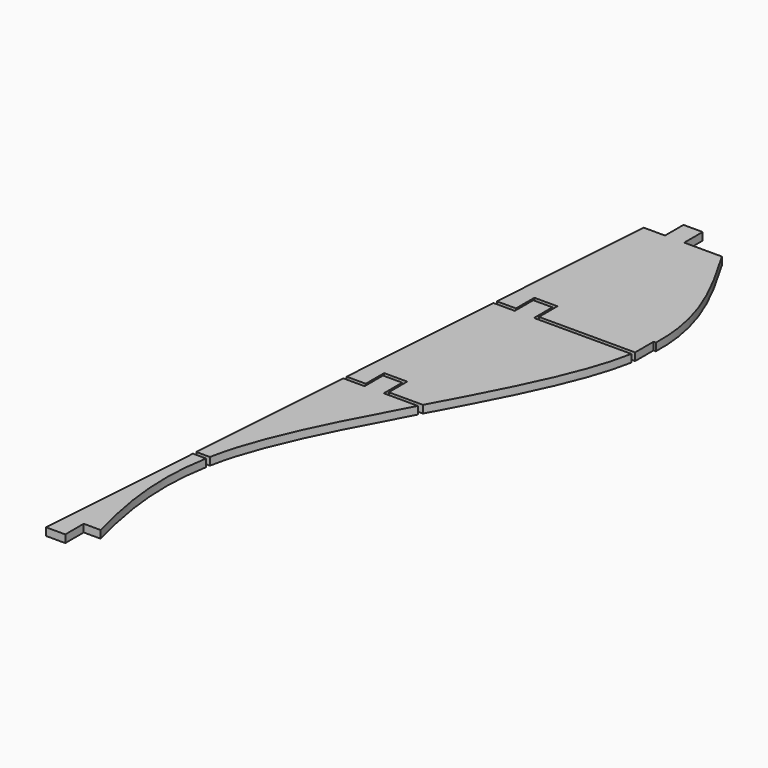
from build123d import *

# Parameters (mm, degrees)
F1_DEPTH = 2


with BuildPart() as f1:
    # F0 (on Top) → F1 (new body)
    with BuildSketch(Plane.XY):
        with BuildLine():
            Line((-20.4571957112, 87.1), (-23.5168766766, 43.1))
            Line((-23.5168766766, 43.1), (-18.5168766766, 43.1))
            Line((-18.5168766766, 43.1), (-18.5168766766, 49.1))
            Line((-18.5168766766, 49.1), (-12.5168766766, 49.1))
            Line((-12.5168766766, 49.1), (-12.5168766766, 43.1))
            Line((-12.5168766766, 43.1), (12.5168766766, 43.1))
            Line((12.5168766766, 43.1), (12.5168766766, 49.1))
            Line((12.5168766766, 49.1), (13.1200117893, 49.0999999996))
            add(Edge.make_bspline(
                [(-0.0691957112, 87.1), (6.7670600664, 75.385477326), (13.603315844, 63.6709546521), (13.1200117893, 49.0999999996)],
                knots=[0, 0, 0, 0, 0.2539558406, 0.2539558406, 0.2539558406, 0.2539558406], degree=3))
            Line((-0.0691957112, 87.1), (-9.8876575074, 87.1))
            Line((-9.8876575074, 87.1), (-9.8876575074, 93.1))
            Line((-9.8876575074, 93.1), (-14.8876575074, 93.1))
            Line((-14.8876575074, 93.1), (-14.8876575074, 87.1))
            Line((-14.8876575074, 87.1), (-20.4571957112, 87.1))
        make_face()
    extrude(amount=F1_DEPTH)


with BuildPart() as f1b:
    # F0 (on Top) → F1, piece 2 (new body)
    with BuildSketch(Plane.XY):
        with BuildLine():
            add(Edge.make_bspline(
                [(-26.4305470242, -47.9), (-28.9813165577, -61.9153804796), (-26.6038291609, -74.0441530198), (-23.513396984, -85.9)],
                knots=[0.7330193554, 0.7330193554, 0.7330193554, 0.7330193554, 0.9613773268, 0.9613773268, 0.9613773268, 0.9613773268], degree=3))
            Line((-26.4305470242, -47.9), (-29.8448532186, -47.9))
            Line((-29.8448532186, -47.9), (-32.904534184, -91.9))
            Line((-32.904534184, -91.9), (-27.904534184, -91.9))
            Line((-27.904534184, -91.9), (-27.904534184, -85.9))
            Line((-27.904534184, -85.9), (-23.513396984, -85.9))
        make_face()
    extrude(amount=F1_DEPTH)


with BuildPart() as f1c:
    # F0 (on Top) → F1, piece 3 (new body)
    with BuildSketch(Plane.XY):
        with BuildLine():
            add(Edge.make_bspline(
                [(-7.2735192987, -2.9), (-14.3461911795, -16.0313284972), (-22.5779302826, -31.4336846167), (-25.8532730678, -44.9386606326), (-26.2407663034, -46.9)],
                knots=[0.5130445245, 0.5130445245, 0.5130445245, 0.5130445245, 0.6958534771, 0.7276056207, 0.7276056207, 0.7276056207, 0.7276056207], degree=3))
            Line((-7.2735192987, -2.9), (-16.1460958457, -2.9))
            Line((-16.1460958457, -2.9), (-16.1460958457, 3.1))
            Line((-16.1460958457, 3.1), (-21.1460958457, 3.1))
            Line((-21.1460958457, 3.1), (-21.1460958457, -2.9))
            Line((-21.1460958457, -2.9), (-26.7156340495, -2.9))
            Line((-26.7156340495, -2.9), (-29.7753150149, -46.9))
            Line((-29.7753150149, -46.9), (-26.2407663034, -46.9))
        make_face()
    extrude(amount=F1_DEPTH)


with BuildPart() as f1d:
    # F0 (on Top) → F1, piece 4 (new body)
    with BuildSketch(Plane.XY):
        with BuildLine():
            add(Edge.make_bspline(
                [(12.3391092449, 42.1), (9.8637373658, 28.9555074487), (1.5856940975, 13.5460464111), (-6.7348489575, -1.9)],
                knots=[0.2933629272, 0.2933629272, 0.2933629272, 0.2933629272, 0.5084039656, 0.5084039656, 0.5084039656, 0.5084039656], degree=3))
            Line((12.3391092449, 42.1), (-13.0168766766, 42.1))
            Line((-13.0168766766, 42.1), (-13.0168766766, 48.1))
            Line((-13.0168766766, 48.1), (-18.0168766766, 48.1))
            Line((-18.0168766766, 48.1), (-18.0168766766, 42.1))
            Line((-18.0168766766, 42.1), (-23.5864148803, 42.1))
            Line((-23.5864148803, 42.1), (-26.6460958457, -1.9))
            Line((-26.6460958457, -1.9), (-21.6460958457, -1.9))
            Line((-21.6460958457, -1.9), (-21.6460958457, 4.1))
            Line((-21.6460958457, 4.1), (-15.6460958457, 4.1))
            Line((-15.6460958457, 4.1), (-15.6460958457, -1.9))
            Line((-15.6460958457, -1.9), (-6.7348489575, -1.9))
        make_face()
    extrude(amount=F1_DEPTH)


solid = Compound([f1.part, f1b.part, f1c.part, f1d.part])
